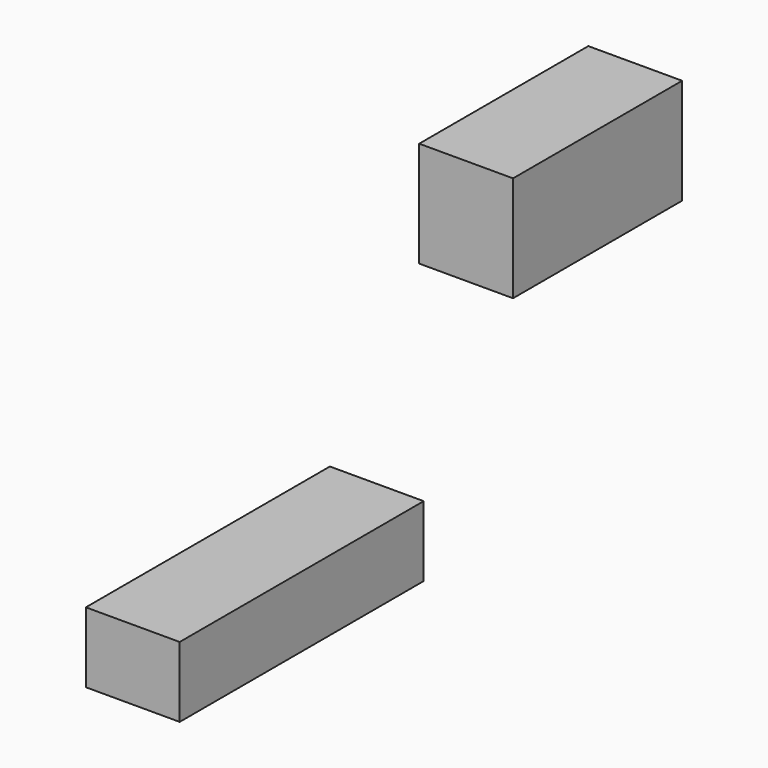
from build123d import *

# Parameters (mm, degrees)
F0_W     = 82.55
F0_H     = 19.05
F1_DEPTH = 25.4


# Not quite as in the source:
# - the program builds the solid bodies; features that only make, move or delete a surface that nothing else refers to are left out


with BuildPart() as f1:
    # F0 (on Right) → F1 (new body)
    with BuildSketch(Plane.YZ):
        with Locations((3.6226294778, -5.7332926338)):
            Rectangle(F0_W, F0_H)
    extrude(amount=-F1_DEPTH)


with BuildPart() as f1b:
    # F0 (on Right) → F1, piece 2 (new body)
    with BuildSketch(Plane.YZ):
        Polygon((75.1320355881, 68.4194193109), (75.1320355881, 49.7785689481), (75.1320355881, 39.8444193109), (132.3449026117, 39.8444193109), (132.3449026117, 68.4194193109), align=None)
    extrude(amount=-F1_DEPTH)


solid = Compound([f1.part, f1b.part])
